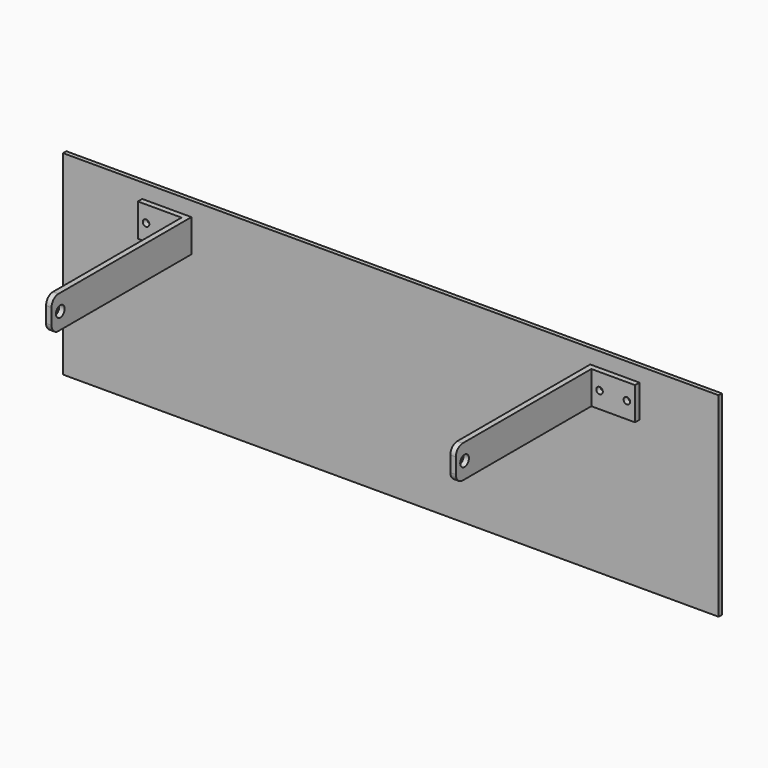
from build123d import *

# Parameters (mm, degrees)
F1_DEPTH  = 2.38125
F3_DEPTH  = 101.6
F5_DEPTH  = 25000
F6_R      = 5
F7_R      = 5
F8_R      = 5
F9_R      = 1.905
F10_DEPTH = 3.175


# Not quite as in the source:
# - a length typed as a fraction of an inch, garbled in the dataset ("3 / 203.2 mm" for 3/8 in), is restored


with BuildPart() as f1:
    # F0 (on Front) → F1 (new body)
    with BuildSketch(Plane.XZ):
        Polygon((190.5, -36), (190.5, 36), (-190.5, 36), (-190.5, -36), (-190.5, -77.319), (190.5, -77.319), align=None)
    extrude(amount=F1_DEPTH)


with BuildPart() as f3:
    # F2 (on face) → F3 (new body)
    with BuildSketch(Plane.XZ.offset(2.38125)):
        Polygon((115.8875, 27.525), (115.8875, 18), (115.8875, 8.475), (119.0625, 8.475), (119.0625, 18), (119.0625, 27.525), align=None)
    extrude(amount=F3_DEPTH)


with BuildPart() as f3b:
    # F2 (on face) → F3, piece 2 (new body)
    with BuildSketch(Plane.XZ.offset(2.38125)):
        Polygon((-115.8875, 8.475), (-115.8875, 18), (-115.8875, 27.525), (-119.0625, 27.525), (-119.0625, 18), (-119.0625, 8.475), align=None)
    extrude(amount=F3_DEPTH)


with BuildPart() as f5_tool:
    # F4 (on face) → F5 (new body)
    with BuildSketch(Plane(origin=(-119.0625, 0, 0), x_dir=(0, -1, 0), z_dir=(-1, 0, 0))):
        with BuildLine():
            ThreePointArc((94.45625, 18), (97.63125, 14.825), (100.80625, 18))
            ThreePointArc((100.80625, 18), (97.63125, 21.175), (94.45625, 18))
        make_face()
    extrude(amount=-F5_DEPTH)


with BuildPart() as f3_1:
    add(f3.part)

    # F5: cut by f5_tool
    add(f5_tool.part, mode=Mode.SUBTRACT)

    # F8
    f8_edges = [f3_1.edges().sort_by_distance(p)[0] for p in [
        (117.475, -103.98125, 27.525),
        (117.475, -103.98125, 8.475),
    ]]
    fillet(f8_edges, radius=F8_R)

    # F9 (on face) → F10, piece 2 (join)
    with BuildSketch(Plane.XZ.offset(2.38125)):
        Polygon((119.0625, 18), (119.0625, 8.475), (131.7625, 8.475), (131.7625, 18), (131.7625, 27.525), (119.0625, 27.525), align=None)
        with Locations((123.825, 18)):
            Circle(F9_R, mode=Mode.SUBTRACT)
        Polygon((131.7625, 18), (131.7625, 8.475), (144.4625, 8.475), (144.4625, 27.525), (131.7625, 27.525), align=None)
        with BuildLine():
            ThreePointArc((141.605, 18), (139.7, 16.095), (137.795, 18))
            ThreePointArc((137.795, 18), (139.7, 19.905), (141.605, 18))
        make_face(mode=Mode.SUBTRACT)
    extrude(amount=F10_DEPTH)


with BuildPart() as f3b_1:
    add(f3b.part)

    # F5: cut by f5_tool
    add(f5_tool.part, mode=Mode.SUBTRACT)

    # F6
    f6_edges = [f3b_1.edges().sort_by_distance(p)[0] for p in [
        (-117.475, -103.98125, 27.525),
    ]]
    fillet(f6_edges, radius=F6_R)

    # F7
    f7_edges = [f3b_1.edges().sort_by_distance(p)[0] for p in [
        (-117.475, -103.98125, 8.475),
    ]]
    fillet(f7_edges, radius=F7_R)

    # F9 (on face) → F10 (join)
    with BuildSketch(Plane.XZ.offset(2.38125)):
        Polygon((-131.7625, 8.475), (-119.0625, 8.475), (-119.0625, 18), (-119.0625, 27.525), (-131.7625, 27.525), (-131.7625, 18), align=None)
        with BuildLine():
            ThreePointArc((-121.92, 18), (-123.825, 16.095), (-125.73, 18))
            ThreePointArc((-125.73, 18), (-123.825, 19.905), (-121.92, 18))
        make_face(mode=Mode.SUBTRACT)
        Polygon((-144.4625, 8.475), (-131.7625, 8.475), (-131.7625, 18), (-131.7625, 27.525), (-144.4625, 27.525), align=None)
        with Locations((-139.7, 18)):
            Circle(F9_R, mode=Mode.SUBTRACT)
    extrude(amount=F10_DEPTH)


solid = Compound([f1.part, f3_1.part, f3b_1.part])
